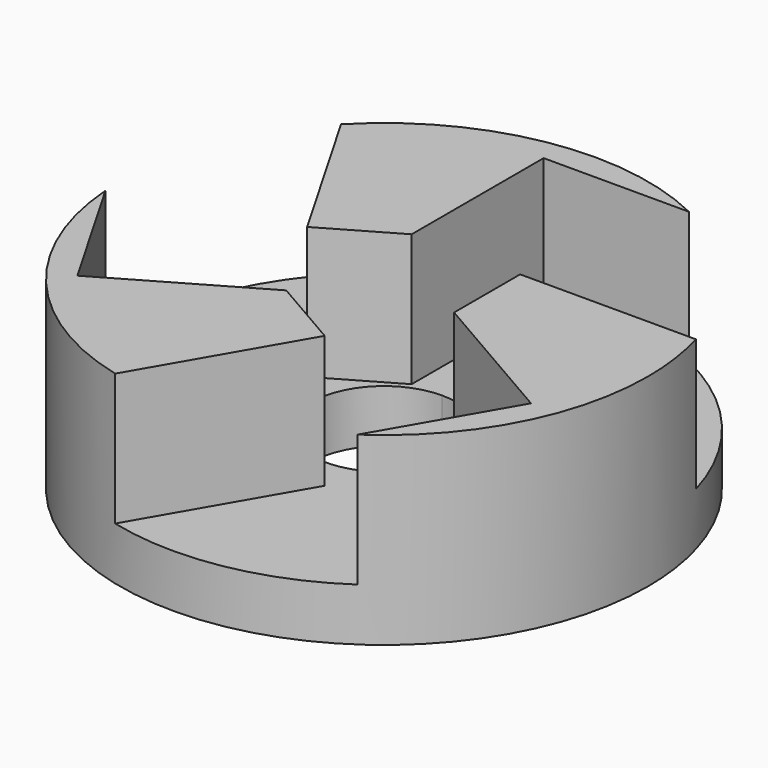
from build123d import *

# Parameters (mm, degrees)
F1_DEPTH = 2
F2_DEPTH = 7


# Not quite as in the source:
# - a feature names something its author has since deleted; it is built from what else it names


with BuildPart() as f1:
    # F0 (on Top) → F1 (new body)
    with BuildSketch(Plane.XY):
        with BuildLine():
            Line((2.9579698818, 2.75), (9.6144422615, 2.75))
            ThreePointArc((9.6144422615, 2.75), (7.6537044043, 6.4359000064), (4.3588989435, 9))
            Line((4.3588989435, 9), (-1.1528000428, 9))
            Line((-1.1528000428, 9), (-1.1528000428, 2.75))
            Line((-1.1528000428, 2.75), (0, 2.75))
            Line((0, 2.75), (2.9579698818, 2.75))
        make_face()
        with BuildLine():
            ThreePointArc((-2.4256512704, -9.7013512417), (1.7468006996, -9.8462524503), (5.6147791623, -8.2749172176))
            Line((5.6147791623, -8.2749172176), (8.3706286555, -3.5016458774))
            Line((8.3706286555, -3.5016458774), (2.9579698818, -0.3766458774))
            Line((2.9579698818, -0.3766458774), (2.3815698685, -1.3749999859))
            Line((2.3815698685, -1.3749999859), (0.9025849195, -3.9366770613))
            Line((0.9025849195, -3.9366770613), (-2.4256512704, -9.7013512417))
        make_face()
        with BuildLine():
            Line((2.9579698818, -0.3766458774), (2.9579698818, 2.75))
            Line((2.9579698818, 2.75), (0, 2.75))
            ThreePointArc((0, 2.75), (1.9445436483, 1.9445436483), (2.75, 0))
            ThreePointArc((2.75, 0), (2.6562960244, -0.7117523662), (2.3815698685, -1.3749999859))
            Line((2.3815698685, -1.3749999859), (2.9579698818, -0.3766458774))
        make_face()
        with BuildLine():
            Line((-3.8605548013, 1.1866770613), (-7.1887909912, 6.9513512417))
            ThreePointArc((-7.1887909912, 6.9513512417), (-9.4005051039, 3.410352444), (-9.9736781058, -0.7250827824))
            Line((-9.9736781058, -0.7250827824), (-7.2178286127, -5.4983541226))
            Line((-7.2178286127, -5.4983541226), (-1.805169839, -2.3733541226))
            Line((-1.805169839, -2.3733541226), (-2.3815698389, -1.3750000373))
            Line((-2.3815698389, -1.3750000373), (-3.8605548013, 1.1866770613))
        make_face()
        with BuildLine():
            ThreePointArc((-2.3815698389, -1.3750000373), (-2.3815698712, 1.3749999814), (0, 2.75))
            Line((0, 2.75), (-1.1528000428, 2.75))
            Line((-1.1528000428, 2.75), (-3.8605548013, 1.1866770613))
            Line((-3.8605548013, 1.1866770613), (-2.3815698389, -1.3750000373))
        make_face()
        with BuildLine():
            Line((-1.805169839, -2.3733541226), (0.9025849195, -3.9366770613))
            Line((0.9025849195, -3.9366770613), (2.3815698685, -1.3749999859))
            ThreePointArc((2.3815698685, -1.3749999859), (2.97e-08, -2.75), (-2.3815698389, -1.3750000373))
            Line((-2.3815698389, -1.3750000373), (-1.805169839, -2.3733541226))
        make_face()
    extrude(amount=F1_DEPTH)

    # F0 (on Top) → F2 (join)
    with BuildSketch(Plane.XY):
        with BuildLine():
            Line((-1.1528000428, 9), (4.3588989435, 9))
            ThreePointArc((4.3588989435, 9), (-1.7468006996, 9.8462524503), (-7.1887909912, 6.9513512417))
            Line((-7.1887909912, 6.9513512417), (-3.8605548013, 1.1866770613))
            Line((-3.8605548013, 1.1866770613), (-1.1528000428, 2.75))
            Line((-1.1528000428, 2.75), (-1.1528000428, 9))
        make_face()
        with BuildLine():
            ThreePointArc((5.6147791623, -8.2749172176), (8.8359434025, -4.6825318139), (10, 0))
            ThreePointArc((10, 0), (9.9031414868, 1.3884483038), (9.6144422615, 2.75))
            Line((9.6144422615, 2.75), (2.9579698818, 2.75))
            Line((2.9579698818, 2.75), (2.9579698818, -0.3766458774))
            Line((2.9579698818, -0.3766458774), (8.3706286555, -3.5016458774))
            Line((8.3706286555, -3.5016458774), (5.6147791623, -8.2749172176))
        make_face()
        with BuildLine():
            ThreePointArc((-9.9736781058, -0.7250827824), (-7.6537044043, -6.4359000064), (-2.4256512704, -9.7013512417))
            Line((-2.4256512704, -9.7013512417), (0.9025849195, -3.9366770613))
            Line((0.9025849195, -3.9366770613), (-1.805169839, -2.3733541226))
            Line((-1.805169839, -2.3733541226), (-7.2178286127, -5.4983541226))
            Line((-7.2178286127, -5.4983541226), (-9.9736781058, -0.7250827824))
        make_face()
    extrude(amount=F2_DEPTH)


solid = f1.part
